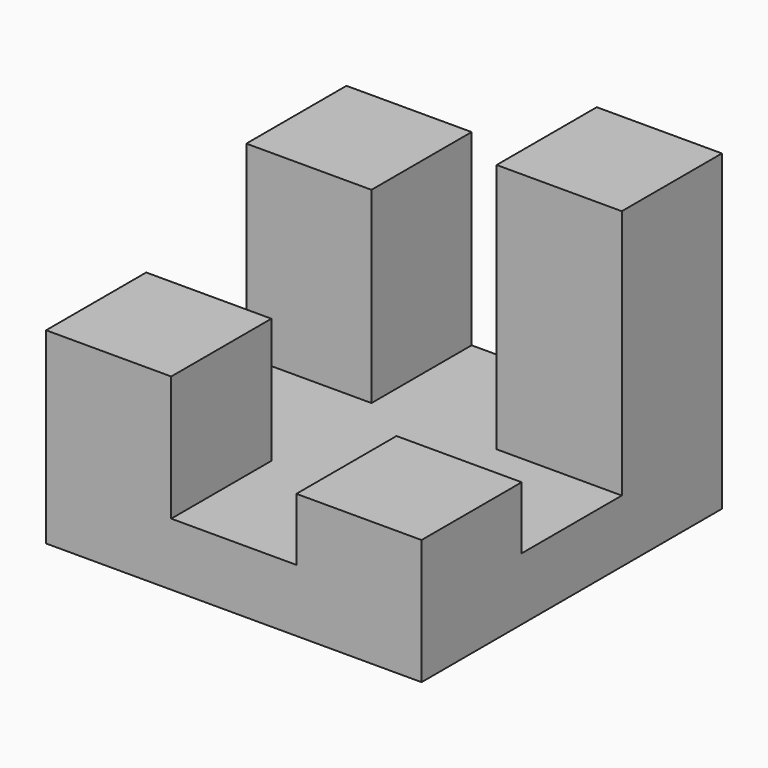
from build123d import *

# Parameters (mm, degrees)
F0_W     = 76.2
F0_H     = 76.2
F1_DEPTH = 12.7
F2_W     = 25.4
F2_H     = 25.4
F3_DEPTH = 12.7
F4_DEPTH = 12.7
F5_DEPTH = 25.4
F6_DEPTH = 38.1


with BuildPart() as f1:
    # F0 (on Top) → F1 (new body)
    with BuildSketch(Plane.XY):
        with Locations((9.7960191858, -9.8835891113)):
            Rectangle(F0_W, F0_H)
    extrude(amount=F1_DEPTH)

    # F2 (on face) → F3 (join)
    with BuildSketch(Plane.XY.offset(12.7)):
        with Locations((35.1960191858, -35.2835891113)):
            Rectangle(F2_W, F2_H)
        with Locations((-15.6039808142, -35.2835891113)):
            Rectangle(F2_W, F2_H)
        with Locations((-15.6039808142, 15.5164108887)):
            Rectangle(F2_W, F2_H)
        with Locations((35.1960191858, 15.5164108887)):
            Rectangle(F2_W, F2_H)
    extrude(amount=F3_DEPTH)

    # F4 (add): a face of the model
    f4_faces = [f1.faces().sort_by_distance(p)[0] for p in [
        (-15.6039808142, -35.2835891113, 25.4),
    ]]
    extrude(f4_faces, amount=F4_DEPTH)

    # F5 (add): a face of the model
    f5_faces = [f1.faces().sort_by_distance(p)[0] for p in [
        (-15.6039808142, 15.5164108887, 25.4),
    ]]
    extrude(f5_faces, amount=F5_DEPTH)

    # F6 (add): a face of the model
    f6_faces = [f1.faces().sort_by_distance(p)[0] for p in [
        (35.1960191858, 15.5164108887, 25.4),
    ]]
    extrude(f6_faces, amount=F6_DEPTH)


solid = f1.part
